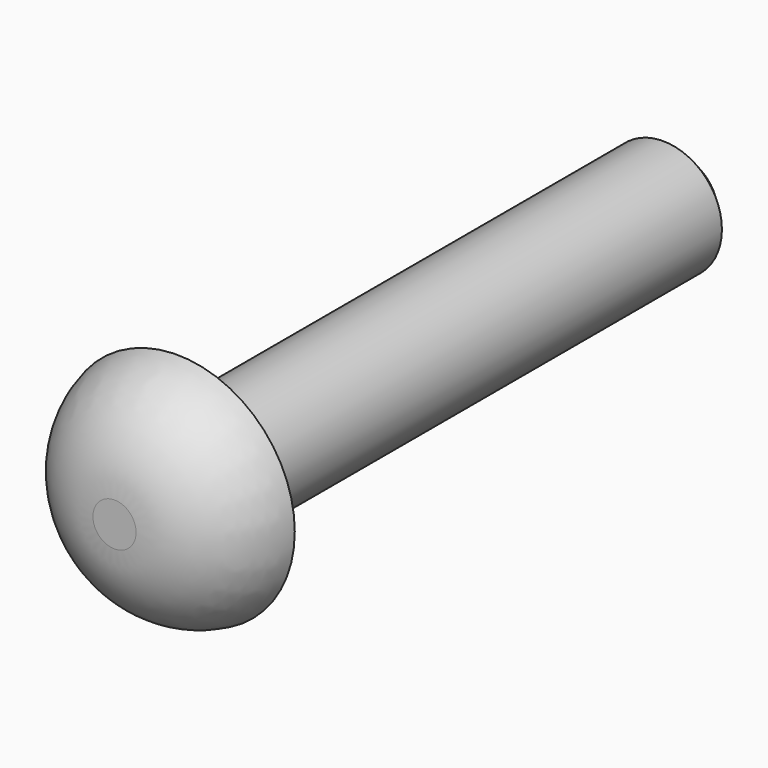
from build123d import *

# Parameters (mm, degrees)
F0_R     = 1.5
F1_DEPTH = 16
F0_R_2   = 3
F2_DEPTH = 2
F4_SIZE  = 0.5


# Not quite as in the source:
# - a fillet or chamfer that OpenCascade refuses, or shapes differently, is made with other operations: its cross-section is extruded or revolved along the edge and cut away or added


with BuildPart() as f1:
    # F0 (on Front) → F1 (new body)
    with BuildSketch(Plane.XZ):
        Circle(F0_R)
    extrude(amount=-F1_DEPTH)

    # F0 (on Front) → F2 (join)
    with BuildSketch(Plane.XZ):
        Circle(F0_R_2)
        Circle(F0_R, mode=Mode.SUBTRACT)
        Circle(F0_R)
    extrude(amount=F2_DEPTH)

    # F3: fillet of radius 2.5 on 1 edges, made by hand

    # F3_s1 → F3_t2 (revolve, cut)
    with BuildSketch(Plane.XY):
        with BuildLine():
            ThreePointArc((3, 0), (2.1316490873, -1.4364916731), (0.5505102572, -2))
            Line((0.5505102572, -2), (3, -2))
            Line((3, -2), (3, 0))
        make_face()
    revolve(axis=Axis((0, -2, 0), (0, -1, 0)), mode=Mode.SUBTRACT)

    # F4
    f4_edges = [f1.edges().sort_by_distance(p)[0] for p in [
        (-1.5, 16, 0),
    ]]
    chamfer(f4_edges, length=F4_SIZE)


solid = f1.part
